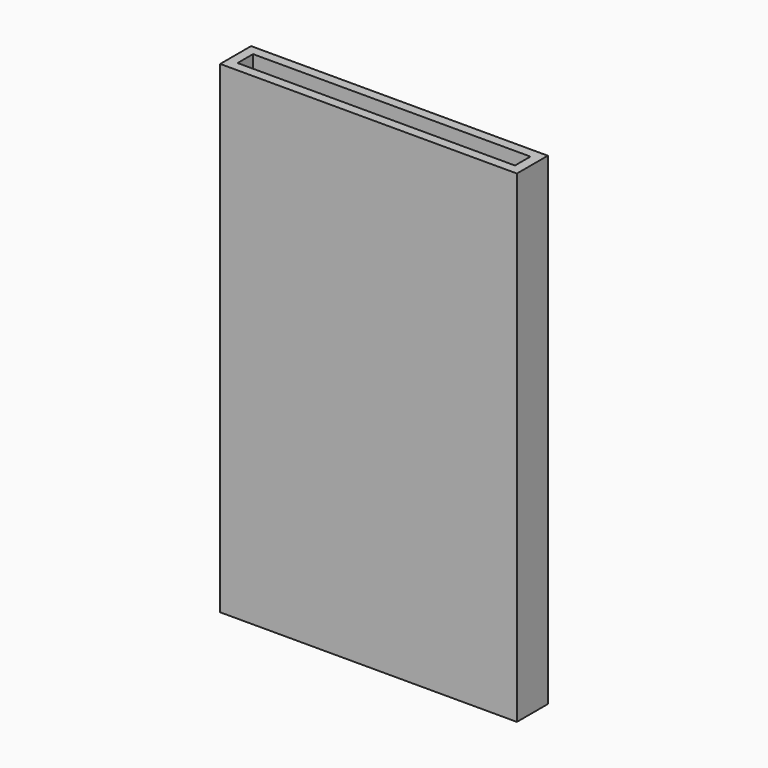
from build123d import *

# Parameters (mm, degrees)
F0_W     = 78.0542
F0_H     = 127
F1_DEPTH = 10.16
F2_T     = -7.62
F3_T     = -2.54


with BuildPart() as f1:
    # F0 (on Front) → F1 (new body)
    with BuildSketch(Plane.XZ):
        Rectangle(F0_W, F0_H)
    extrude(amount=F1_DEPTH)

    # F2
    f2_openings = [f1.faces().sort_by_distance(p)[0] for p in [
        (0, 0, 0),
    ]]
    offset(amount=F2_T, openings=f2_openings)

    # F3
    f3_openings = [f1.faces().sort_by_distance(p)[0] for p in [
        (0, -5.08, 63.5),
    ]]
    offset(amount=F3_T, openings=f3_openings, kind=Kind.INTERSECTION)


solid = f1.part
